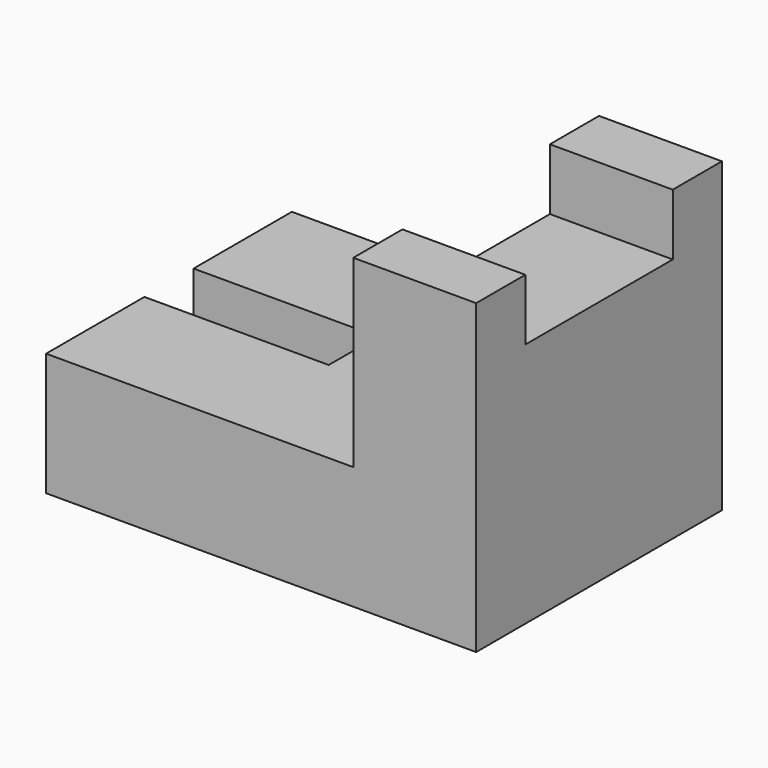
from build123d import *

# Parameters (mm, degrees)
F1_DEPTH = 31.75
F2_W     = 19.05
F2_H     = 6.35
F3_DEPTH = 25.4
F4_W     = 6.35
F4_H     = 12.7
F5_DEPTH = 19.05


# Not quite as in the source:
# - a feature names something its author has since deleted; it is built from what else it names


with BuildPart() as f1:
    # F0 (on Front) → F1 (new body)
    with BuildSketch(Plane.XZ):
        Polygon((0, 12.7), (0, 0), (44.45, 0), (44.45, 12.7), (44.45, 31.75), (31.75, 31.75), (31.75, 12.7), align=None)
    extrude(amount=F1_DEPTH)

    # F2 (on face) → F3 (cut)
    with BuildSketch(Plane(origin=(31.75, 0, 0), x_dir=(0, -1, 0), z_dir=(-1, 0, 0))):
        with Locations((15.875, 28.575)):
            Rectangle(F2_W, F2_H)
    extrude(amount=-F3_DEPTH, mode=Mode.SUBTRACT)

    # F4 (on face) → F5 (cut)
    with BuildSketch(Plane(origin=(0, 0, 0), x_dir=(0, -1, 0), z_dir=(-1, 0, 0))):
        with Locations((15.875, 6.35)):
            Rectangle(F4_W, F4_H)
    extrude(amount=-F5_DEPTH, mode=Mode.SUBTRACT)


solid = f1.part
